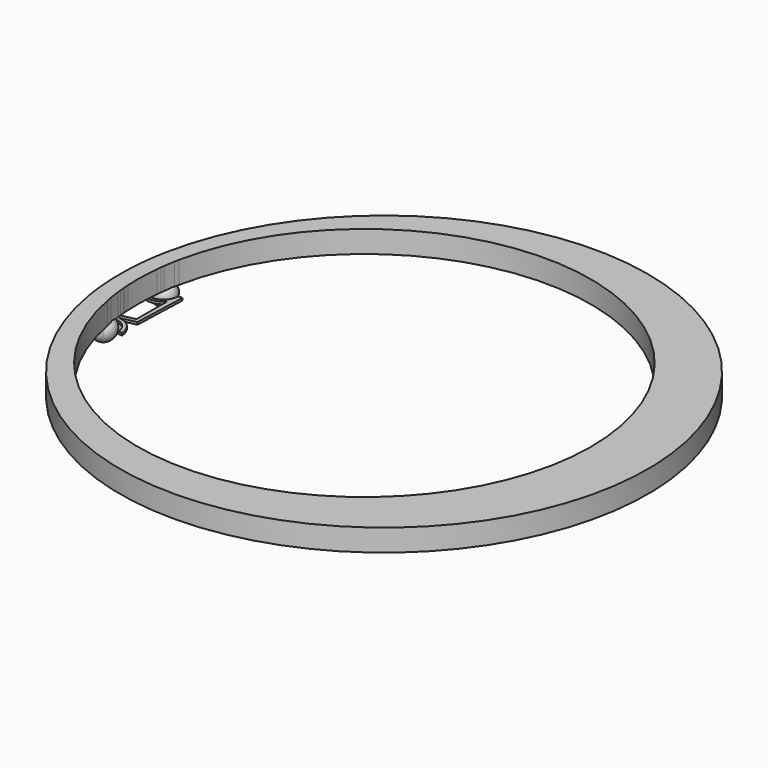
from build123d import *

# Parameters (mm, degrees)
F1_DEPTH      = 1
F1_DEPTH_BACK = 1
F3_START      = 6.25
F3_DEPTH      = 18.75


with BuildPart() as f1:
    # F0 (on Top) → F1 (new body, two sides)
    with BuildSketch(Plane.XY) as f1_sk:
        with BuildLine():
            ThreePointArc((5.3003190322, -17.9200269408), (5.4519181466, -19.6345637583), (5.6188172673, -21.3476788955))
            ThreePointArc((5.6188172673, -21.3476788955), (10.6352454567, -25.9720916376), (12.5284092501, -32.5269124468))
            Line((12.5284092501, -32.5269124468), (15.8096607774, -32.5269124468))
            ThreePointArc((15.8096607774, -32.5269124468), (12.8354231694, -23.5827467282), (5.3003190322, -17.9200269408))
        make_face()
        with BuildLine():
            ThreePointArc((0, -19.9604799519), (2.8896243917, -20.3291673494), (5.6188172673, -21.3476788955))
            ThreePointArc((5.6188172673, -21.3476788955), (5.4519181466, -19.6345637583), (5.3003190322, -17.9200269408))
            ThreePointArc((5.3003190322, -17.9200269408), (2.689341962, -17.2356052448), (0, -17.0052270113))
            Line((0, -17.0052270113), (0, -19.9604799519))
        make_face()
        with BuildLine():
            ThreePointArc((-8.3388992418, -22.9597984106), (-4.440045657, -20.7078105735), (0, -19.9604799519))
            Line((0, -19.9604799519), (0, -17.0052270113))
            ThreePointArc((0, -17.0052270113), (-4.4915370969, -17.6565584493), (-8.6130491677, -19.5568943105))
            ThreePointArc((-8.6130491677, -19.5568943105), (-8.4824430271, -21.2588675116), (-8.3388992418, -22.9597984106))
        make_face()
        with BuildLine():
            ThreePointArc((-12.8267044201, -32.5269124468), (-11.6271072761, -27.2534857181), (-8.3388992418, -22.9597984106))
            ThreePointArc((-8.3388992418, -22.9597984106), (-8.4824430271, -21.2588675116), (-8.6130491677, -19.5568943105))
            ThreePointArc((-8.6130491677, -19.5568943105), (-13.8265155726, -25.1457069814), (-15.8096607774, -32.5269124468))
            Line((-15.8096607774, -32.5269124468), (-12.8267044201, -32.5269124468))
        make_face()
    extrude(amount=F1_DEPTH)
    extrude(f1_sk.sketch, amount=-F1_DEPTH_BACK)


with BuildPart() as f1b:
    # F0 (on Top) → F1, piece 2 (new body, two sides)
    with BuildSketch(Plane.XY) as f1_2_sk:
        with BuildLine():
            Line((-8.881291048, -15.3281712863), (0, -17.0052270113))
            Line((0, -17.0052270113), (0, -13.4232956916))
            Line((0, -13.4232956916), (-9.05574971, -11.4827777524))
            ThreePointArc((-9.05574971, -11.4827777523), (-8.9767627231, -13.4058484598), (-8.881291048, -15.3281712863))
        make_face()
        with BuildLine():
            Line((-15.8096607774, -14.0198860317), (-8.881291048, -15.3281712863))
            ThreePointArc((-8.881291048, -15.3281712863), (-8.9767627231, -13.4058484598), (-9.05574971, -11.4827777523))
            Line((-9.05574971, -11.4827777524), (-12.5284092501, -10.738636367))
            Line((-12.5284092501, -10.738636367), (-12.5284092501, 22.808624168))
            ThreePointArc((-12.5284092501, 22.808624168), (-14.8830436931, 27.1059194382), (-15.8096607774, 31.917616725))
            Line((-15.8096607774, 31.917616725), (-15.8096607774, -14.0198860317))
        make_face()
        with BuildLine():
            Line((-12.8267044201, 31.917616725), (-15.8096607774, 31.917616725))
            ThreePointArc((-15.8096607774, 31.917616725), (-14.8830436931, 27.1059194382), (-12.5284092501, 22.808624168))
            ThreePointArc((-12.5284092501, 22.808624168), (-10.5062256605, 20.6405878581), (-8.1150247047, 18.8879424577))
            ThreePointArc((-8.1150247047, 18.8879424577), (-7.9626512783, 20.3762433144), (-7.8003626904, 21.8634956518))
            ThreePointArc((-7.8003626904, 21.8634956518), (-11.504380015, 26.2952180966), (-12.8267044201, 31.917616725))
        make_face()
        with BuildLine():
            ThreePointArc((-8.1150247047, 18.8879424577), (-4.2092582578, 17.2181895505), (0, 16.6478990731))
            Line((0, 16.6478990731), (0, 19.3725855164))
            ThreePointArc((0, 19.3725855164), (-4.1094291672, 19.9627745105), (-7.8003626904, 21.8634956518))
            ThreePointArc((-7.8003626904, 21.8634956518), (-7.9626512783, 20.3762433144), (-8.1150247047, 18.8879424577))
        make_face()
        with BuildLine():
            Line((0, 19.3725855164), (0, 16.6478990731))
            ThreePointArc((0, 16.6478990731), (2.8521073568, 16.9071319802), (5.6107384631, 17.6763344853))
            ThreePointArc((5.6107384631, 17.6763344853), (5.7900143917, 19.3680441711), (5.9842097449, 21.0581062067))
            ThreePointArc((5.9842097449, 21.0581062067), (3.0983174718, 19.8382526132), (0, 19.3725855164))
        make_face()
        with BuildLine():
            ThreePointArc((11.0369324684, 21.1342585721), (14.4656522663, 26.0645896884), (15.8096607774, 31.917616725))
            Line((15.8096607774, 31.917616725), (12.23011408, 31.917616725))
            ThreePointArc((12.23011408, 31.917616725), (10.5619472354, 25.6511340701), (5.9842097449, 21.0581062067))
            ThreePointArc((5.9842097449, 21.0581062067), (5.7900143917, 19.3680441711), (5.6107384631, 17.6763344853))
            ThreePointArc((5.6107384631, 17.6763344853), (8.5015026089, 19.1265002444), (11.0369324684, 21.1342585721))
        make_face()
        with BuildLine():
            ThreePointArc((4.914580284, -12.3606835702), (5.0206899204, -14.1433284216), (5.1433060929, -15.9249140063))
            Line((5.1433060929, -15.9249140063), (14.2130312032, -14.0198860317))
            Line((14.2130312032, -14.0198860317), (15.8096607774, 31.917616725))
            ThreePointArc((15.8096607774, 31.917616725), (14.4656522663, 26.0645896884), (11.0369324684, 21.1342585721))
            Line((11.0369324684, 21.1342585721), (11.0369324684, -11.0369315371))
            Line((11.0369324684, -11.0369315371), (4.914580284, -12.3606835702))
        make_face()
        with BuildLine():
            Line((0, -13.4232956916), (0, -17.0052270113))
            Line((0, -17.0052270113), (5.1433060929, -15.9249140063))
            ThreePointArc((5.1433060929, -15.9249140063), (5.0206899204, -14.1433284216), (4.914580284, -12.3606835702))
            Line((4.914580284, -12.3606835702), (0, -13.4232956916))
        make_face()
    extrude(amount=F1_DEPTH)
    extrude(f1_2_sk.sketch, amount=-F1_DEPTH_BACK)


with BuildPart() as f2:
    # F0 (on Top) → F2 (revolve)
    with BuildSketch(Plane.XY):
        with BuildLine():
            ThreePointArc((8.1234616975, -38.3586677614), (9.5193123957, -35.5900303865), (10, -32.5269124468))
            ThreePointArc((10, -32.5269124468), (8.9349292743, -28.0361398113), (5.9665922274, -24.5019652698))
            ThreePointArc((5.9665922274, -24.5019652698), (6.531492286, -28.8432959991), (7.1948170662, -33.1706814468))
            ThreePointArc((7.1948170662, -33.1706814468), (7.6414114113, -35.767847894), (8.1234616975, -38.3586677614))
        make_face()
        with BuildLine():
            ThreePointArc((7.1948170662, -33.1706814468), (6.531492286, -28.8432959991), (5.9665922274, -24.5019652698))
            ThreePointArc((5.9665922274, -24.5019652698), (3.142493296, -23.0335075842), (0, -22.5269124468))
            Line((0, -22.5269124468), (0, -42.5269124468))
            ThreePointArc((0, -42.5269124468), (4.5652188805, -41.4240342608), (8.1234616975, -38.3586677614))
            ThreePointArc((8.1234616975, -38.3586677614), (7.6414114113, -35.767847894), (7.1948170662, -33.1706814468))
        make_face()
        with BuildLine():
            ThreePointArc((-7.2877490893, -32.5269124468), (-7.6621150003, -29.5266586158), (-7.9960391137, -26.5216348935))
            ThreePointArc((-7.9960391137, -26.5216348935), (-9.908679156, -33.8752734454), (-6.1006233613, -40.4504466711))
            ThreePointArc((-6.1006233613, -40.4504466711), (-6.7295376984, -36.493976014), (-7.2877490893, -32.5269124468))
        make_face()
    revolve(axis=Axis((0, -0.3046478609, 0), (0, 1, 0)))


with BuildPart() as f2b:
    # F0 (on Top) → F2, piece 2 (revolve)
    with BuildSketch(Plane.XY):
        with BuildLine():
            ThreePointArc((10, 31.917616725), (9.6383902497, 34.5824682021), (8.5797133209, 37.0545924239))
            ThreePointArc((8.5797133209, 37.0545924239), (8.1934646149, 35.1273427272), (7.8268833458, 33.1962555647))
            ThreePointArc((7.8268833458, 33.1962555647), (7.0549966282, 28.718887232), (6.3888255555, 24.2245738926))
            ThreePointArc((6.3888255555, 24.2245738926), (9.0522995851, 27.6683965351), (10, 31.917616725))
        make_face()
        with BuildLine():
            Line((0, 21.917616725), (0, 41.917616725))
            ThreePointArc((0, 41.917616725), (-2.5199788975, 41.5948945631), (-4.8773071875, 40.6475579962))
            ThreePointArc((-4.8773071875, 40.6475579962), (-5.6038490401, 36.8301460552), (-6.264204625, 33.0007299781))
            ThreePointArc((-6.264204625, 33.0007299781), (-6.8667625523, 29.1015177407), (-7.4006996933, 25.1923179175))
            ThreePointArc((-7.4006996933, 25.1923179175), (-4.046418906, 22.7728644573), (0, 21.917616725))
        make_face()
        with BuildLine():
            ThreePointArc((-6.264204625, 33.0007299781), (-5.6038490401, 36.8301460552), (-4.8773071875, 40.6475579962))
            ThreePointArc((-4.8773071875, 40.6475579962), (-9.8693198709, 33.5289904514), (-7.4006996933, 25.1923179175))
            ThreePointArc((-7.4006996933, 25.1923179175), (-6.8667625523, 29.1015177407), (-6.264204625, 33.0007299781))
        make_face()
    revolve(axis=Axis((0, -0.3046478609, 0), (0, 1, 0)))


with BuildPart() as f3:
    # F0 (on Top) → F3 (new body)
    with BuildSketch(Plane.XY.offset(F3_START)):
        with BuildLine():
            ThreePointArc((7.1948170662, -33.1706814468), (6.531492286, -28.8432959991), (5.9665922274, -24.5019652698))
            ThreePointArc((5.9665922274, -24.5019652698), (3.142493296, -23.0335075842), (0, -22.5269124468))
            Line((0, -22.5269124468), (0, -42.5269124468))
            ThreePointArc((0, -42.5269124468), (4.5652188805, -41.4240342608), (8.1234616975, -38.3586677614))
            ThreePointArc((8.1234616975, -38.3586677614), (7.6414114113, -35.767847894), (7.1948170662, -33.1706814468))
        make_face()
        with BuildLine():
            ThreePointArc((0, -22.5269124468), (3.142493296, -23.0335075842), (5.9665922274, -24.5019652698))
            ThreePointArc((5.9665922274, -24.5019652698), (5.7862150263, -22.9255376051), (5.6188172673, -21.3476788955))
            ThreePointArc((5.6188172673, -21.3476788955), (2.8896243917, -20.3291673494), (0, -19.9604799519))
            Line((0, -19.9604799519), (0, -22.5269124468))
        make_face()
        with BuildLine():
            ThreePointArc((390.2340564281, -1.7959624641), (215.7943387416, -193.7239033847), (8.1234616975, -38.3586677614))
            ThreePointArc((8.1234616975, -38.3586677614), (4.5652188805, -41.4240342608), (0, -42.5269124468))
            ThreePointArc((0, -42.5269124468), (-3.2221621434, -41.9935734802), (-6.1006233613, -40.4504466711))
            ThreePointArc((-6.1006233613, -40.4504466711), (233.955821601, -226.942723079), (439.7708302282, -3.2316412089))
            ThreePointArc((439.7708302282, -3.2316412089), (237.3278649488, 220.1723371745), (-4.8773071875, 40.6475579962))
            ThreePointArc((-4.8773071875, 40.6475579962), (-2.5199788975, 41.5948945631), (0, 41.917616725))
            ThreePointArc((0, 41.917616725), (4.9310365549, 40.6173223806), (8.5797133209, 37.0545924239))
            ThreePointArc((8.5797133209, 37.0545924239), (216.9551490026, 190.0173603447), (390.2340564281, -1.7959624641))
        make_face()
        with BuildLine():
            Line((0, -42.5269124468), (0, -22.5269124468))
            ThreePointArc((0, -22.5269124468), (-4.4691847393, -23.5811655374), (-7.9960391137, -26.5216348935))
            ThreePointArc((-7.9960391137, -26.5216348935), (-7.6621150003, -29.5266586158), (-7.2877490893, -32.5269124468))
            ThreePointArc((-7.2877490893, -32.5269124468), (-6.7295376984, -36.493976014), (-6.1006233613, -40.4504466711))
            ThreePointArc((-6.1006233613, -40.4504466711), (-3.2221621434, -41.9935734802), (0, -42.5269124468))
        make_face()
        with BuildLine():
            ThreePointArc((-7.9960391137, -26.5216348935), (-4.4691847393, -23.5811655374), (0, -22.5269124468))
            Line((0, -22.5269124468), (0, -19.9604799519))
            ThreePointArc((0, -19.9604799519), (-4.440045657, -20.7078105735), (-8.3388992418, -22.9597984106))
            ThreePointArc((-8.3388992418, -22.9597984106), (-8.1745661374, -24.7413998009), (-7.9960391137, -26.5216348935))
        make_face()
        with BuildLine():
            ThreePointArc((0, -19.9604799519), (2.8896243917, -20.3291673494), (5.6188172673, -21.3476788955))
            ThreePointArc((5.6188172673, -21.3476788955), (5.4519181466, -19.6345637583), (5.3003190322, -17.9200269408))
            ThreePointArc((5.3003190322, -17.9200269408), (2.689341962, -17.2356052448), (0, -17.0052270113))
            Line((0, -17.0052270113), (0, -19.9604799519))
        make_face()
        with BuildLine():
            ThreePointArc((-8.3388992418, -22.9597984106), (-4.440045657, -20.7078105735), (0, -19.9604799519))
            Line((0, -19.9604799519), (0, -17.0052270113))
            ThreePointArc((0, -17.0052270113), (-4.4915370969, -17.6565584493), (-8.6130491677, -19.5568943105))
            ThreePointArc((-8.6130491677, -19.5568943105), (-8.4824430271, -21.2588675116), (-8.3388992418, -22.9597984106))
        make_face()
        with BuildLine():
            ThreePointArc((0, -17.0052270113), (2.689341962, -17.2356052448), (5.3003190322, -17.9200269408))
            ThreePointArc((5.3003190322, -17.9200269408), (5.2192239245, -16.9226741962), (5.1433060929, -15.9249140063))
            Line((5.1433060929, -15.9249140063), (0, -17.0052270113))
        make_face()
        with BuildLine():
            ThreePointArc((7.8268833458, 33.1962555647), (8.1934646149, 35.1273427272), (8.5797133209, 37.0545924239))
            ThreePointArc((8.5797133209, 37.0545924239), (4.9310365549, 40.6173223806), (0, 41.917616725))
            Line((0, 41.917616725), (0, 21.917616725))
            ThreePointArc((0, 21.917616725), (3.3962900109, 22.512021892), (6.3888255555, 24.2245738926))
            ThreePointArc((6.3888255555, 24.2245738926), (7.0549966282, 28.718887232), (7.8268833458, 33.1962555647))
        make_face()
        with BuildLine():
            ThreePointArc((-8.6130491677, -19.5568943105), (-4.4915370969, -17.6565584493), (0, -17.0052270113))
            Line((0, -17.0052270113), (-8.881291048, -15.3281712863))
            ThreePointArc((-8.881291048, -15.3281712863), (-8.7571474494, -17.4431656942), (-8.6130491677, -19.5568943105))
        make_face()
        with BuildLine():
            Line((0, -13.4232956916), (0, -17.0052270113))
            Line((0, -17.0052270113), (5.1433060929, -15.9249140063))
            ThreePointArc((5.1433060929, -15.9249140063), (5.0206899204, -14.1433284216), (4.914580284, -12.3606835702))
            Line((4.914580284, -12.3606835702), (0, -13.4232956916))
        make_face()
        with BuildLine():
            Line((-8.881291048, -15.3281712863), (0, -17.0052270113))
            Line((0, -17.0052270113), (0, -13.4232956916))
            Line((0, -13.4232956916), (-9.05574971, -11.4827777524))
            ThreePointArc((-9.05574971, -11.4827777523), (-8.9767627231, -13.4058484598), (-8.881291048, -15.3281712863))
        make_face()
        with BuildLine():
            Line((0, 21.917616725), (0, 41.917616725))
            ThreePointArc((0, 41.917616725), (-2.5199788975, 41.5948945631), (-4.8773071875, 40.6475579962))
            ThreePointArc((-4.8773071875, 40.6475579962), (-5.6038490401, 36.8301460552), (-6.264204625, 33.0007299781))
            ThreePointArc((-6.264204625, 33.0007299781), (-6.8667625523, 29.1015177407), (-7.4006996933, 25.1923179175))
            ThreePointArc((-7.4006996933, 25.1923179175), (-4.046418906, 22.7728644573), (0, 21.917616725))
        make_face()
        with BuildLine():
            Line((0, 16.6478990731), (0, -13.4232956916))
            Line((0, -13.4232956916), (4.914580284, -12.3606835702))
            ThreePointArc((4.914580284, -12.3606835702), (4.676678319, 2.6714065495), (5.6107384631, 17.6763344853))
            ThreePointArc((5.6107384631, 17.6763344853), (2.8521073568, 16.9071319802), (0, 16.6478990731))
        make_face()
        with BuildLine():
            Line((-9.05574971, -11.4827777524), (0, -13.4232956916))
            Line((0, -13.4232956916), (0, 16.6478990731))
            ThreePointArc((0, 16.6478990731), (-4.2092582578, 17.2181895505), (-8.1150247047, 18.8879424577))
            ThreePointArc((-8.1150247047, 18.8879424577), (-9.0998230799, 3.7185168674), (-9.05574971, -11.4827777523))
        make_face()
        with BuildLine():
            ThreePointArc((5.9842097449, 21.0581062067), (6.1799642421, 22.6421774536), (6.3888255555, 24.2245738926))
            ThreePointArc((6.3888255555, 24.2245738926), (3.3962900109, 22.512021892), (0, 21.917616725))
            Line((0, 21.917616725), (0, 19.3725855164))
            ThreePointArc((0, 19.3725855164), (3.0983174718, 19.8382526132), (5.9842097449, 21.0581062067))
        make_face()
        with BuildLine():
            Line((0, 19.3725855164), (0, 21.917616725))
            ThreePointArc((0, 21.917616725), (-4.046418906, 22.7728644573), (-7.4006996933, 25.1923179175))
            ThreePointArc((-7.4006996933, 25.1923179175), (-7.6067457425, 23.5286529122), (-7.8003626904, 21.8634956518))
            ThreePointArc((-7.8003626904, 21.8634956518), (-4.1094291672, 19.9627745105), (0, 19.3725855164))
        make_face()
        with BuildLine():
            Line((0, 19.3725855164), (0, 16.6478990731))
            ThreePointArc((0, 16.6478990731), (2.8521073568, 16.9071319802), (5.6107384631, 17.6763344853))
            ThreePointArc((5.6107384631, 17.6763344853), (5.7900143917, 19.3680441711), (5.9842097449, 21.0581062067))
            ThreePointArc((5.9842097449, 21.0581062067), (3.0983174718, 19.8382526132), (0, 19.3725855164))
        make_face()
        with BuildLine():
            ThreePointArc((-8.1150247047, 18.8879424577), (-4.2092582578, 17.2181895505), (0, 16.6478990731))
            Line((0, 16.6478990731), (0, 19.3725855164))
            ThreePointArc((0, 19.3725855164), (-4.1094291672, 19.9627745105), (-7.8003626904, 21.8634956518))
            ThreePointArc((-7.8003626904, 21.8634956518), (-7.9626512783, 20.3762433144), (-8.1150247047, 18.8879424577))
        make_face()
    extrude(amount=F3_DEPTH)


solid = Compound([f1.part, f1b.part, f2.part, f2b.part, f3.part])
